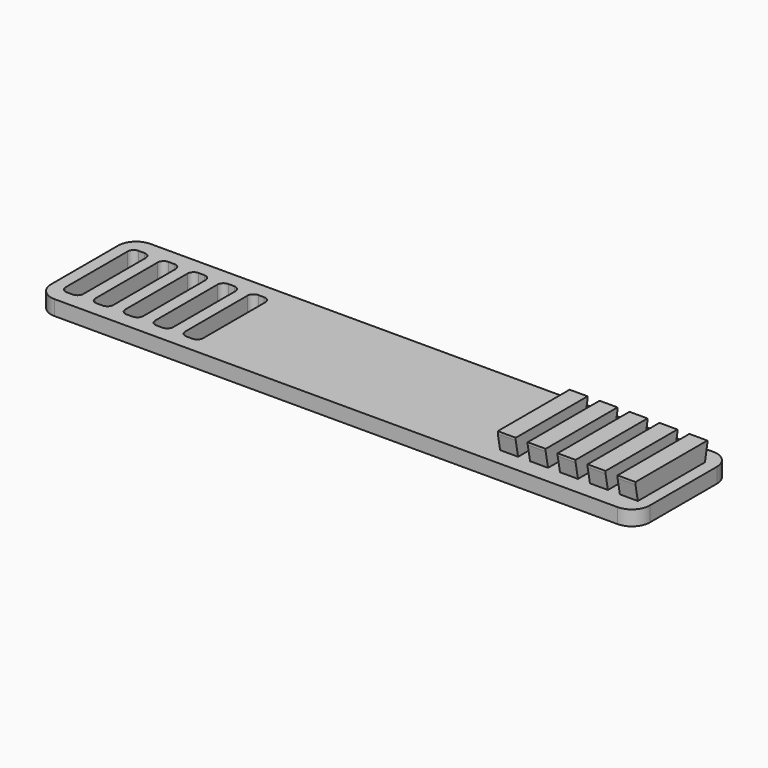
from build123d import *

# Parameters (mm, degrees)
F0_W     = 100
F0_H     = 20
F0_W_2   = 3
F0_H_2   = 15
F1_DEPTH = 2.5
F2_W     = 3
F2_H     = 15
F3_DEPTH = 3
F5_DEPTH = 98.001
F6_R     = 3


# Not quite as in the source:
# - a feature names something its author has since deleted; it is built from what else it names


with BuildPart() as f1:
    # F0 (on Top) → F1 (new body)
    with BuildSketch(Plane.XY):
        Rectangle(F0_W, F0_H)
        with BuildLine():
            ThreePointArc((-45, -6.5), (-45.2928932188, -7.2071067812), (-46, -7.5))
            Line((-46, -7.5), (-47, -7.5))
            ThreePointArc((-47, -7.5), (-47.7071067812, -7.2071067812), (-48, -6.5))
            Line((-48, -6.5), (-48, 6.5))
            ThreePointArc((-48, 6.5), (-47.7071067812, 7.2071067812), (-47, 7.5))
            Line((-47, 7.5), (-46, 7.5))
            ThreePointArc((-46, 7.5), (-45.2928932188, 7.2071067812), (-45, 6.5))
            Line((-45, 6.5), (-45, -6.5))
        make_face(mode=Mode.SUBTRACT)
        with BuildLine():
            Line((-42, 7.5), (-41, 7.5))
            ThreePointArc((-41, 7.5), (-40.2928932188, 7.2071067812), (-40, 6.5))
            Line((-40, 6.5), (-40, -6.5))
            ThreePointArc((-40, -6.5), (-40.2928932188, -7.2071067812), (-41, -7.5))
            Line((-41, -7.5), (-42, -7.5))
            ThreePointArc((-42, -7.5), (-42.7071067812, -7.2071067812), (-43, -6.5))
            Line((-43, -6.5), (-43, 6.5))
            ThreePointArc((-43, 6.5), (-42.7071067812, 7.2071067812), (-42, 7.5))
        make_face(mode=Mode.SUBTRACT)
        with BuildLine():
            Line((-37, 7.5), (-36, 7.5))
            ThreePointArc((-36, 7.5), (-35.2928932188, 7.2071067812), (-35, 6.5))
            Line((-35, 6.5), (-35, -6.5))
            ThreePointArc((-35, -6.5), (-35.2928932188, -7.2071067812), (-36, -7.5))
            Line((-36, -7.5), (-37, -7.5))
            ThreePointArc((-37, -7.5), (-37.7071067812, -7.2071067812), (-38, -6.5))
            Line((-38, -6.5), (-38, 6.5))
            ThreePointArc((-38, 6.5), (-37.7071067812, 7.2071067812), (-37, 7.5))
        make_face(mode=Mode.SUBTRACT)
        with BuildLine():
            Line((-32, 7.5), (-31, 7.5))
            ThreePointArc((-31, 7.5), (-30.2928932188, 7.2071067812), (-30, 6.5))
            Line((-30, 6.5), (-30, -6.5))
            ThreePointArc((-30, -6.5), (-30.2928932188, -7.2071067812), (-31, -7.5))
            Line((-31, -7.5), (-32, -7.5))
            ThreePointArc((-32, -7.5), (-32.7071067812, -7.2071067812), (-33, -6.5))
            Line((-33, -6.5), (-33, 6.5))
            ThreePointArc((-33, 6.5), (-32.7071067812, 7.2071067812), (-32, 7.5))
        make_face(mode=Mode.SUBTRACT)
        with BuildLine():
            Line((-27, 7.5), (-26, 7.5))
            ThreePointArc((-26, 7.5), (-25.2928932188, 7.2071067812), (-25, 6.5))
            Line((-25, 6.5), (-25, -6.5))
            ThreePointArc((-25, -6.5), (-25.2928932188, -7.2071067812), (-26, -7.5))
            Line((-26, -7.5), (-27, -7.5))
            ThreePointArc((-27, -7.5), (-27.7071067812, -7.2071067812), (-28, -6.5))
            Line((-28, -6.5), (-28, 6.5))
            ThreePointArc((-28, 6.5), (-27.7071067812, 7.2071067812), (-27, 7.5))
        make_face(mode=Mode.SUBTRACT)
        with Locations((26.5, 0)):
            Rectangle(F0_W_2, F0_H_2, mode=Mode.SUBTRACT)
        with Locations((31.5, 0)):
            Rectangle(F0_W_2, F0_H_2, mode=Mode.SUBTRACT)
        with Locations((36.5, 0)):
            Rectangle(F0_W_2, F0_H_2, mode=Mode.SUBTRACT)
        with Locations((41.5, 0)):
            Rectangle(F0_W_2, F0_H_2, mode=Mode.SUBTRACT)
        with Locations((46.5, 0)):
            Rectangle(F0_W_2, F0_H_2, mode=Mode.SUBTRACT)
        with Locations((26.5, 0)):
            Rectangle(F0_W_2, F0_H_2)
        with Locations((31.5, 0)):
            Rectangle(F0_W_2, F0_H_2)
        with Locations((36.5, 0)):
            Rectangle(F0_W_2, F0_H_2)
        with Locations((41.5, 0)):
            Rectangle(F0_W_2, F0_H_2)
        with Locations((46.5, 0)):
            Rectangle(F0_W_2, F0_H_2)
    extrude(amount=F1_DEPTH)

    # F2 (on face) → F3 (join)
    with BuildSketch(Plane.XY.offset(2.5)):
        with Locations((26.5, 0)):
            Rectangle(F2_W, F2_H)
        with Locations((31.5, 0)):
            Rectangle(F2_W, F2_H)
        with Locations((36.5, 0)):
            Rectangle(F2_W, F2_H)
        with Locations((41.5, 0)):
            Rectangle(F2_W, F2_H)
        with Locations((46.5, 0)):
            Rectangle(F2_W, F2_H)
    extrude(amount=F3_DEPTH)

    # F4 (on face) → F5 (cut, through all)
    with BuildSketch(Plane.YZ.offset(48)):
        Polygon((-7.5, 5.1), (-7.5, 2.5), (-7, 2.5), align=None)
        Polygon((7.5, 5.1), (7, 2.5), (7.5, 2.5), align=None)
    extrude(amount=-F5_DEPTH, mode=Mode.SUBTRACT)

    # F6
    f6_edges = [f1.edges().sort_by_distance(p)[0] for p in [
        (-50, -10, 1.25),
        (50, -10, 1.25),
        (-50, 10, 1.25),
        (50, 10, 1.25),
    ]]
    fillet(f6_edges, radius=F6_R)


solid = f1.part
